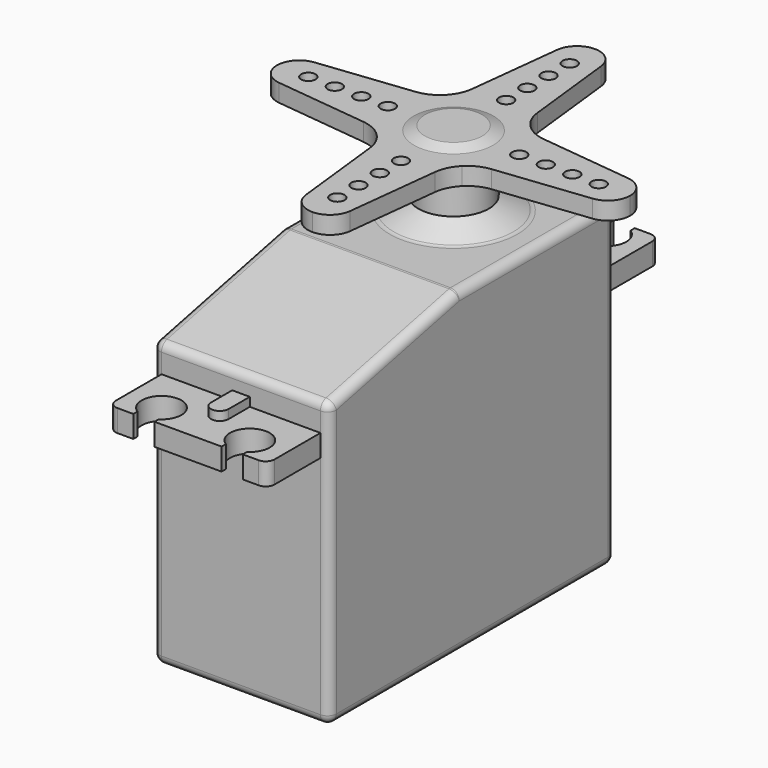
from build123d import *

# Parameters (mm, degrees)
F1_DEPTH  = 10
F0_W      = 7.5
F0_H      = 2.5
F2_DEPTH  = 9
F4_DEPTH  = 25
F5_W      = 2
F5_H      = 46.5
F6_DEPTH  = 1
F9_R      = 0.8128
F10_DEPTH = 2
F11_R     = 26.294756744
F12_DEPTH = 2
F13_R     = 0.99999


# Not quite as in the source:
# - a fillet or chamfer is up to 0.001 mm smaller than in the source, because OpenCascade refuses the exact size


with BuildPart() as f1:
    # F0 (on Right) → F1 (new body, symmetric)
    with BuildSketch(Plane.YZ):
        Polygon((-20.25, 26.6), (-20.25, 0), (20.25, 0), (20.25, 26.6), (20.25, 29.1), (20.25, 36.1), (-1.95, 36.1), (-20.25, 32.1), (-20.25, 29.1), align=None)
    extrude(amount=F1_DEPTH, both=True)

    # F0 (on Right) → F2 (join, symmetric)
    with BuildSketch(Plane.YZ):
        with Locations((-24, 27.85)):
            Rectangle(F0_W, F0_H)
        with Locations((24, 27.85)):
            Rectangle(F0_W, F0_H)
    extrude(amount=F2_DEPTH, both=True)

    # F3 (on face) → F4 (cut)
    with BuildSketch(Plane.XY.offset(29.1)):
        with BuildLine():
            ThreePointArc((-3.8, -27.1532866311), (-3.0299111695, -26.336853256), (-2.75, -25.25))
            ThreePointArc((-2.75, -25.25), (-6.086853256, -23.2799111695), (-6.2, -27.1532866311))
            ThreePointArc((-6.2, -27.1532866311), (-5, -27.5), (-3.8, -27.1532866311))
        make_face()
        with BuildLine():
            ThreePointArc((-3.8, -27.1532866311), (-5, -27.5), (-6.2, -27.1532866311))
            Line((-6.2, -27.1532866311), (-6.2, -27.75))
            Line((-6.2, -27.75), (-3.8, -27.75))
            Line((-3.8, -27.75), (-3.8, -27.1532866311))
        make_face()
        with BuildLine():
            Line((-3.8, 27.75), (-6.2, 27.75))
            Line((-6.2, 27.75), (-6.2, 27.1532866311))
            ThreePointArc((-6.2, 27.1532866311), (-5, 27.5), (-3.8, 27.1532866311))
            Line((-3.8, 27.1532866311), (-3.8, 27.75))
        make_face()
        with BuildLine():
            ThreePointArc((-3.8, 27.1532866311), (-5, 27.5), (-6.2, 27.1532866311))
            ThreePointArc((-6.2, 27.1532866311), (-6.086853256, 23.2799111695), (-2.75, 25.25))
            ThreePointArc((-2.75, 25.25), (-3.0299111695, 26.336853256), (-3.8, 27.1532866311))
        make_face()
        with BuildLine():
            Line((3.8, -27.1532866311), (3.8, -27.75))
            Line((3.8, -27.75), (6.2, -27.75))
            Line((6.2, -27.75), (6.2, -27.1532866311))
            ThreePointArc((6.2, -27.1532866311), (5, -27.5), (3.8, -27.1532866311))
        make_face()
        with BuildLine():
            ThreePointArc((7.25, -25.25), (3.913146744, -23.2799111695), (3.8, -27.1532866311))
            ThreePointArc((3.8, -27.1532866311), (5, -27.5), (6.2, -27.1532866311))
            ThreePointArc((6.2, -27.1532866311), (6.9700888305, -26.336853256), (7.25, -25.25))
        make_face()
        with BuildLine():
            Line((6.2, 27.75), (3.8, 27.75))
            Line((3.8, 27.75), (3.8, 27.1532866311))
            ThreePointArc((3.8, 27.1532866311), (5, 27.5), (6.2, 27.1532866311))
            Line((6.2, 27.1532866311), (6.2, 27.75))
        make_face()
        with BuildLine():
            ThreePointArc((6.2, 27.1532866311), (5, 27.5), (3.8, 27.1532866311))
            ThreePointArc((3.8, 27.1532866311), (3.913146744, 23.2799111695), (7.25, 25.25))
            ThreePointArc((7.25, 25.25), (6.9700888305, 26.336853256), (6.2, 27.1532866311))
        make_face()
    extrude(amount=-F4_DEPTH, mode=Mode.SUBTRACT)

    # F5 (on face) → F6 (join)
    with BuildSketch(Plane.XY.offset(29.1)):
        Rectangle(F5_W, F5_H)
        with BuildLine():
            Line((-1, 23.25), (1, 23.25))
            ThreePointArc((1, 23.25), (0, 24.25), (-1, 23.25))
        make_face()
        with BuildLine():
            ThreePointArc((-1, -23.25), (0, -24.25), (1, -23.25))
            Line((1, -23.25), (-1, -23.25))
        make_face()
    extrude(amount=F6_DEPTH)

    # F7 (on Right) → F8 (revolve)
    with BuildSketch(Plane.YZ):
        Polygon((9.85, 36.1), (16.85, 36.1), (13.85, 37.6), (13.85, 42.1), (29.85, 42.1), (29.85, 44.1), (14.35, 44.1), (13.1, 44.6), (9.85, 44.6), align=None)
    revolve(axis=Axis((0, 9.85, 38.956922479), (0, 0, -1)))

    # F9 (on face) → F10 (cut, through all)
    with BuildSketch(Plane.XY.offset(44.1)):
        with Locations((0, 17.3)):
            Circle(F9_R)
        with Locations((0, 20.3)):
            Circle(F9_R)
        with Locations((0, 23.3)):
            Circle(F9_R)
        with Locations((0, 26.3)):
            Circle(F9_R)
        with Locations((-16.45, 9.85)):
            Circle(F9_R)
        with Locations((-13.45, 9.85)):
            Circle(F9_R)
        with Locations((-10.45, 9.85)):
            Circle(F9_R)
        with Locations((-7.45, 9.85)):
            Circle(F9_R)
        with Locations((0, -6.6)):
            Circle(F9_R)
        with Locations((0, -3.6)):
            Circle(F9_R)
        with Locations((0, -0.6)):
            Circle(F9_R)
        with Locations((0, 2.4)):
            Circle(F9_R)
        with Locations((16.45, 9.85)):
            Circle(F9_R)
        with Locations((13.45, 9.85)):
            Circle(F9_R)
        with Locations((10.45, 9.85)):
            Circle(F9_R)
        with Locations((7.45, 9.85)):
            Circle(F9_R)
    extrude(amount=-F10_DEPTH, mode=Mode.SUBTRACT)

    # F11 (on face) → F12 (cut, through all)
    with BuildSketch(Plane.XY.offset(44.1)):
        with Locations((0, 9.85)):
            Circle(F11_R)
        with BuildLine():
            ThreePointArc((-4.8436814511, 14.6936814511), (-4.0616110554, 15.7958081166), (-3.6873277698, 17.0943570425))
            Line((-3.6873277698, 17.0943570425), (-2.5, 27.6162423281))
            ThreePointArc((-2.5, 27.6162423281), (-1.6762811024, 29.2102108544), (0, 29.85))
            ThreePointArc((0, 29.85), (1.6762811024, 29.2102108544), (2.5, 27.6162423281))
            Line((2.5, 27.6162423281), (3.6873277698, 17.0943570425))
            ThreePointArc((3.6873277698, 17.0943570425), (4.0616110554, 15.7958081166), (4.8436814511, 14.6936814511))
            ThreePointArc((4.8436814511, 14.6936814511), (5.9458081166, 13.9116110554), (7.2443570425, 13.5373277698))
            Line((7.2443570425, 13.5373277698), (17.7662423281, 12.35))
            ThreePointArc((17.7662423281, 12.35), (19.3602108544, 11.5262811024), (20, 9.85))
            ThreePointArc((20, 9.85), (19.3602108544, 8.1737188976), (17.7662423281, 7.35))
            Line((17.7662423281, 7.35), (7.2443570425, 6.1626722302))
            ThreePointArc((7.2443570425, 6.1626722302), (5.9458081166, 5.7883889446), (4.8436814511, 5.0063185489))
            ThreePointArc((4.8436814511, 5.0063185489), (4.0616110554, 3.9041918834), (3.6873277698, 2.6056429575))
            Line((3.6873277698, 2.6056429575), (2.5, -7.9162423281))
            ThreePointArc((2.5, -7.9162423281), (1.6762811024, -9.5102108544), (0, -10.15))
            ThreePointArc((0, -10.15), (-1.6762811024, -9.5102108544), (-2.5, -7.9162423281))
            Line((-2.5, -7.9162423281), (-3.6873277698, 2.6056429575))
            ThreePointArc((-3.6873277698, 2.6056429575), (-4.0616110554, 3.9041918834), (-4.8436814511, 5.0063185489))
            ThreePointArc((-4.8436814511, 5.0063185489), (-5.9458081166, 5.7883889446), (-7.2443570425, 6.1626722302))
            Line((-7.2443570425, 6.1626722302), (-17.7662423281, 7.35))
            ThreePointArc((-17.7662423281, 7.35), (-19.3602108544, 8.1737188976), (-20, 9.85))
            ThreePointArc((-20, 9.85), (-19.3602108544, 11.5262811024), (-17.7662423281, 12.35))
            Line((-17.7662423281, 12.35), (-7.2443570425, 13.5373277698))
            ThreePointArc((-7.2443570425, 13.5373277698), (-5.9458081166, 13.9116110554), (-4.8436814511, 14.6936814511))
        make_face(mode=Mode.SUBTRACT)
    extrude(amount=-F12_DEPTH, mode=Mode.SUBTRACT)

    # F13 (radius 1 in the source; OpenCascade refuses exactly that, so slightly less here)
    f13_edges = [f1.edges().sort_by_distance(p)[0] for p in [
        (10, -20.25, 16.05),
        (10, 0, 0),
        (10, 20.25, 18.05),
        (10, 9.15, 36.1),
        (10, -11.1, 34.1),
        (-10, 0, 0),
        (-10, 20.25, 18.05),
        (-10, 9.15, 36.1),
        (-10, -11.1, 34.1),
        (-10, -20.25, 16.05),
        (0, -20.25, 0),
        (0, 20.25, 0),
        (0, -1.95, 36.1),
        (0, -20.25, 32.1),
        (0, 20.25, 36.1),
        (0, 2.85, 36.1),
        (9, -27.75, 27.85),
        (-9, -27.75, 27.85),
        (9, 27.75, 27.85),
        (-9, 27.75, 27.85),
    ]]
    fillet(f13_edges, radius=F13_R)


solid = f1.part
